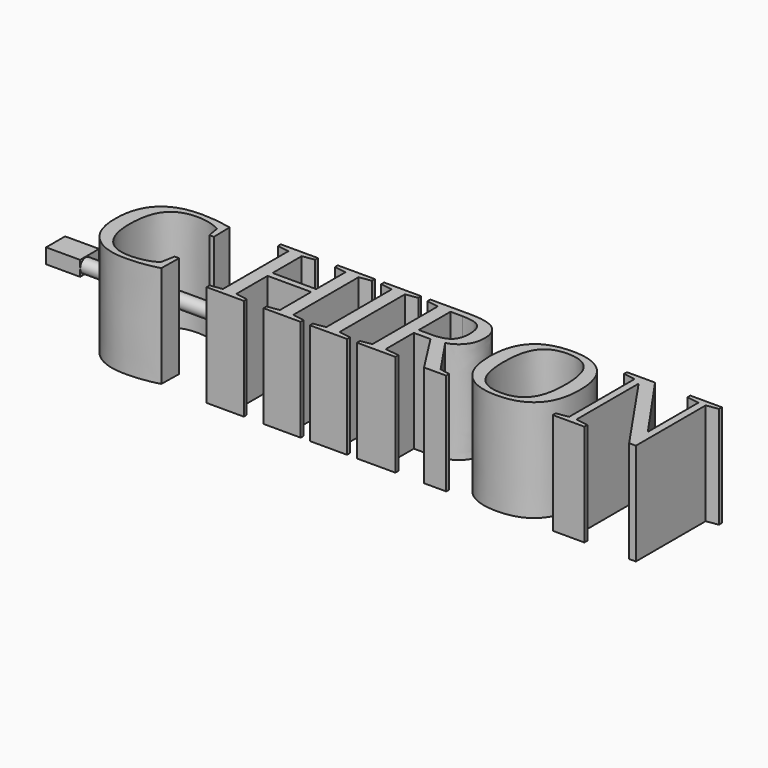
from build123d import *

# Parameters (mm, degrees)
F0_TEXT_SIZE = 26.4583333333
F1_DEPTH     = 19.05
F2_R         = 1.2857096354
F3_DEPTH     = 31.75
F4_W         = 4.445
F4_H         = 2.794
F5_DEPTH     = 6.35


# Not quite as in the source:
# - Text() gives the source's letters only with a copy of the font that has no kerning and outlines rounded to 1/6400 em; it was checked with that copy


with BuildPart() as f1:
    # F0 (on Top) → F1 (new body)
    with BuildSketch(Plane.XY):
        with Locations((0, 0)):
            Text('C HIRON', F0_TEXT_SIZE, font='Tinos', text_align=(TextAlign.LEFT, TextAlign.BOTTOM))
    extrude(amount=F1_DEPTH)


with BuildPart() as f3:
    # F2 (on face) → F3 (new body)
    with BuildSketch(Plane(origin=(27.2479492188, 0, 0), x_dir=(0, -1, 0), z_dir=(-1, 0, 0))):
        with Locations((-8.6692382813, 9.525)):
            Circle(F2_R)
    extrude(amount=F3_DEPTH)


with BuildPart() as f5:
    # F4 (on face) → F5 (new body)
    with BuildSketch(Plane(origin=(-4.5020507812, 0, 0), x_dir=(0, -1, 0), z_dir=(-1, 0, 0))):
        with Locations((-9.5732517505, 9.545864843)):
            Rectangle(F4_W, F4_H)
    extrude(amount=F5_DEPTH)


solid = Compound([f1.part, f3.part, f5.part])
